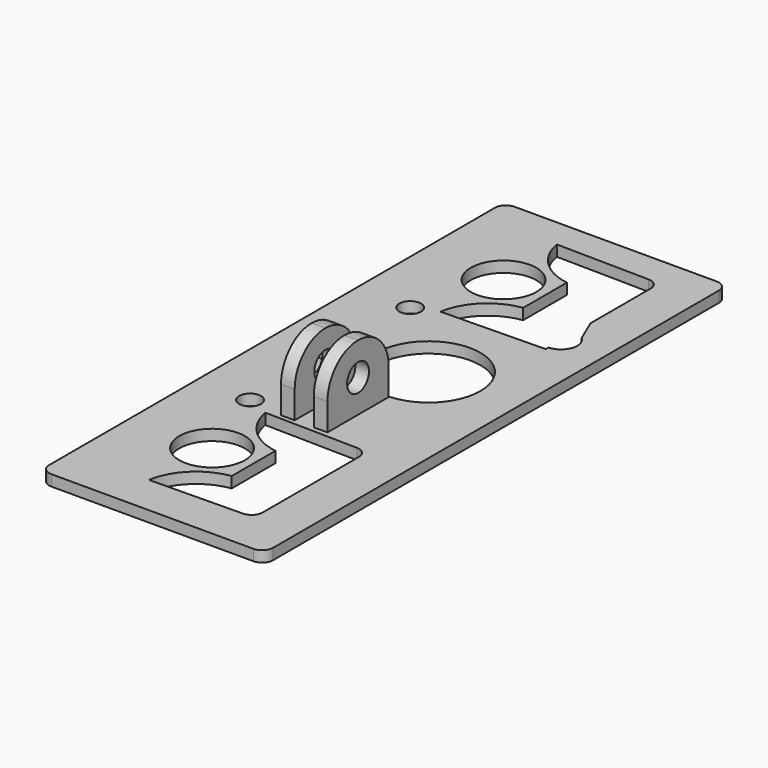
from build123d import *

# Parameters (mm, degrees)
F0_W     = 41
F0_H     = 106
F0_R     = 6
F0_R_2   = 2
F0_W_2   = 2.5
F0_H_2   = 14
F0_R_3   = 9.5
F1_DEPTH = 2
F2_R     = 2
F3_DEPTH = 14
F4_R     = 6.99999
F5_R     = 2.5
F6_DEPTH = 25


# Not quite as in the source:
# - a fillet or chamfer is up to 0.001 mm smaller than in the source, because OpenCascade refuses the exact size


with BuildPart() as f1:
    # F0 (on Top) → F1 (new body)
    with BuildSketch(Plane.XY):
        with Locations((0, 4.2499956787)):
            Rectangle(F0_W, F0_H)
        with Locations((-5.5959895056, -28.0965764523)):
            Circle(F0_R, mode=Mode.SUBTRACT)
        with Locations((-10.6551818848, -13.0636913106)):
            Circle(F0_R_2, mode=Mode.SUBTRACT)
        with Locations((-3, -7)):
            Rectangle(F0_W_2, F0_H_2, mode=Mode.SUBTRACT)
        with BuildLine():
            ThreePointArc((2, -23.0965764523), (-3.6071540429, -20.3211082876), (-6.5, -14.7736005353))
            Line((-6.5, -14.7736005353), (12.5, -15.1310515412))
            Line((12.5, -15.1310515412), (12.5, -41.1310515412))
            Line((12.5, -41.1310515412), (-6.5, -41.4195523692))
            ThreePointArc((-6.5, -41.4195523692), (-3.6071540429, -35.8720446169), (2, -33.0965764523))
            Line((2, -33.0965764523), (2, -23.0965764523))
        make_face(mode=Mode.SUBTRACT)
        with Locations((3, -7)):
            Rectangle(F0_W_2, F0_H_2, mode=Mode.SUBTRACT)
        with Locations((-10.6551818848, 5.2499956787)):
            Circle(F0_R_2, mode=Mode.SUBTRACT)
        with Locations((-10.6551818848, 23.5636826679)):
            Circle(F0_R_2, mode=Mode.SUBTRACT)
        with Locations((-5.5959895056, 38.5965678096)):
            Circle(F0_R, mode=Mode.SUBTRACT)
        with Locations((3.8262721598, 9.6499956787)):
            Circle(F0_R_3, mode=Mode.SUBTRACT)
        with BuildLine():
            ThreePointArc((2, 43.5965678096), (-3.6071540429, 46.3720359742), (-6.5, 51.9195437265))
            Line((-6.5, 51.9195437265), (12.5, 51.6310428985))
            Line((12.5, 51.6310428985), (12.5, 35.8656205144))
            Line((12.5, 35.8656205144), (14.3622287411, 31.5192815504))
            ThreePointArc((14.3622287411, 31.5192815504), (15.1282490927, 30.4976562448), (15.4, 29.2499956787))
            ThreePointArc((15.4, 29.2499956787), (14.5563858653, 27.1643303172), (12.5, 26.2516628086))
            Line((12.5, 26.2516628086), (12.5, 25.6310428985))
            Line((12.5, 25.6310428985), (-6.5, 25.2735918926))
            ThreePointArc((-6.5, 25.2735918926), (-3.6071540429, 30.8210996449), (2, 33.5965678096))
            Line((2, 33.5965678096), (2, 43.5965678096))
        make_face(mode=Mode.SUBTRACT)
    extrude(amount=F1_DEPTH)

    # F2
    f2_edges = [f1.edges().sort_by_distance(p)[0] for p in [
        (20.5, -48.750004, 1),
        (-20.5, -48.750004, 1),
        (12.5, -15.131052, 1),
        (12.5, -41.131052, 1),
        (12.5, 51.631043, 1),
        (20.5, 57.249996, 1),
        (-20.5, 57.249996, 1),
    ]]
    fillet(f2_edges, radius=F2_R)

    # F0 (on Top) → F3 (join)
    with BuildSketch(Plane.XY):
        with Locations((-3, -7)):
            Rectangle(F0_W_2, F0_H_2)
        with Locations((3, -7)):
            Rectangle(F0_W_2, F0_H_2)
    extrude(amount=F3_DEPTH)

    # F4 (radius 7 in the source; OpenCascade refuses exactly that, so slightly less here)
    f4_edges = [f1.edges().sort_by_distance(p)[0] for p in [
        (3, 0, 14),
        (3, -14, 14),
        (-3, -14, 14),
        (-3, 0, 14),
    ]]
    fillet(f4_edges, radius=F4_R)

    # F5 (on face) → F6 (cut)
    with BuildSketch(Plane.YZ.offset(4.25)):
        with Locations((-7, 8)):
            Circle(F5_R)
    extrude(amount=-F6_DEPTH, mode=Mode.SUBTRACT)


solid = f1.part
